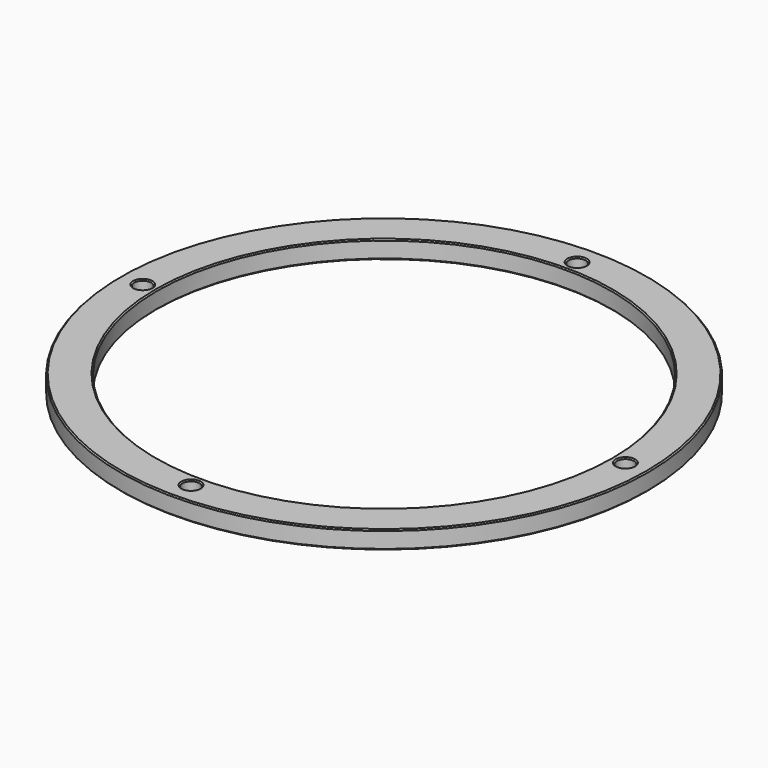
from build123d import *

# Parameters (mm, degrees)
F0_R     = 111.125
F0_R_2   = 95.6945
F1_DEPTH = 7.62
F3_D     = 7.1882
F4_SIZE  = 0.508


with BuildPart() as f1:
    # F0 (on Top) → F1 (new body)
    with BuildSketch(Plane.XY):
        Circle(F0_R)
        Circle(F0_R_2, mode=Mode.SUBTRACT)
    extrude(amount=F1_DEPTH)

    # F3 (through all)
    with Locations(Plane(origin=(0, 0, 0), x_dir=(1, 0, 0), z_dir=(0, 0, -1))):
        with Locations((-101.6, 0), (0, -101.6), (101.6, 0), (0, 101.6)):
            Hole(F3_D / 2)

    # F4
    f4_edges = [f1.edges().sort_by_distance(p)[0] for p in [
        (-111.125, 0, 7.62),
        (-95.6945, 0, 0),
        (-95.6945, 0, 7.62),
        (-111.125, 0, 0),
        (-3.5941, -101.6, 0),
        (-105.1941, 0, 0),
        (98.0059, 0, 0),
        (-3.5941, 101.6, 0),
        (-3.5941, -101.6, 7.62),
        (-105.1941, 0, 7.62),
        (98.0059, 0, 7.62),
        (-3.5941, 101.6, 7.62),
    ]]
    chamfer(f4_edges, length=F4_SIZE)


solid = f1.part
